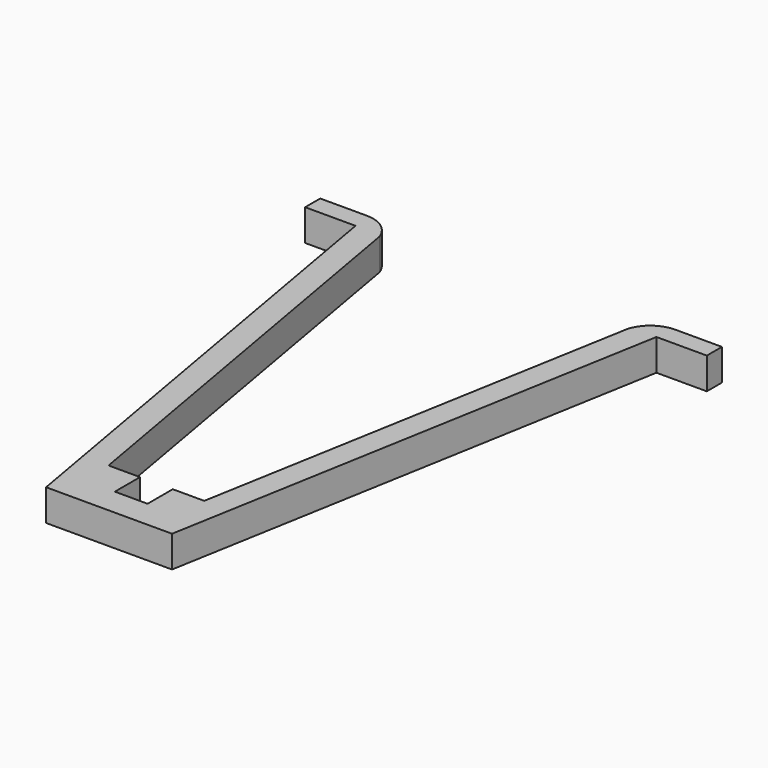
from build123d import *

# Parameters (mm, degrees)
F1_DEPTH    = 5
F2_T1_DEPTH = 28.770290161


# Not quite as in the source:
# - a fillet or chamfer that OpenCascade refuses, or shapes differently, is made with other operations: its cross-section is extruded or revolved along the edge and cut away or added


with BuildPart() as f1:
    # F0 (on Top) → F1 (new body)
    with BuildSketch(Plane.XY):
        Polygon((-10, 0), (0, 0), (10, 0), (23.8918542134, 78.784620241), (31.8918542134, 78.784620241), (31.8918542134, 81.784620241), (19.7553724367, 81.784620241), (19.7553724367, 78.3334689187), (7.6, 9.3969262079), (2.6, 9.3969262079), (2.6, 4.3969262079), (0, 4.3969262079), (-2.6, 4.3969262079), (-2.6, 9.3969262079), (-7.6, 9.3969262079), (-19.7553724367, 78.3334689187), (-19.7553724367, 81.784620241), (-31.8918542134, 81.784620241), (-31.8918542134, 78.784620241), (-23.8918542134, 78.784620241), align=None)
    extrude(amount=F1_DEPTH)

    # F2: fillet of radius 5 on 2 edges, made by hand

    # F2_s2 → F2_t1 (cut)
    with BuildSketch(Plane.XY.offset(-11.8851450805)):
        with BuildLine():
            ThreePointArc((-24.5094304689, 81.784620241), (-21.5721054433, 80.8308680948), (-19.7553724367, 78.3334689187))
            Line((-19.7553724367, 78.3334689187), (-19.7553724367, 81.784620241))
            Line((-19.7553724367, 81.784620241), (-24.5094304689, 81.784620241))
        make_face()
        with BuildLine():
            ThreePointArc((19.7553724367, 78.3334689187), (21.5721054433, 80.8308680948), (24.5094304689, 81.784620241))
            Line((24.5094304689, 81.784620241), (19.7553724367, 81.784620241))
            Line((19.7553724367, 81.784620241), (19.7553724367, 78.3334689187))
        make_face()
    extrude(amount=F2_T1_DEPTH, mode=Mode.SUBTRACT)


solid = f1.part
